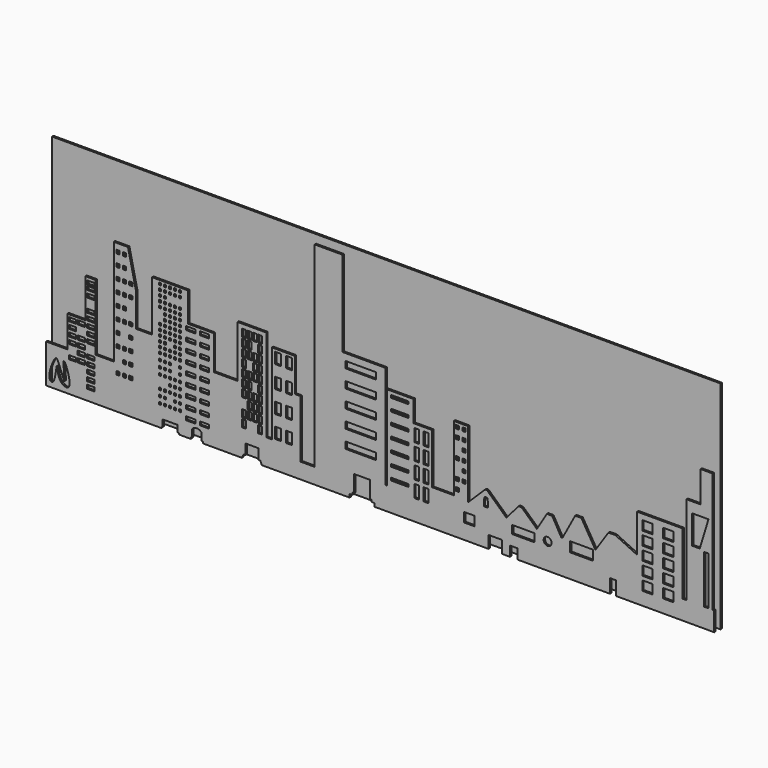
from build123d import *

# Parameters (mm, degrees)
F0_W     = 106.057882309
F0_H     = 53.0289784074
F0_W_2   = 30.3485393524
F0_H_2   = 32.5163006783
F0_W_3   = 133.1057548523
F0_H_3   = 52.0848631859
F0_W_4   = 106.7019701004
F0_H_4   = 55.8841459751
F0_W_5   = 45.7174777985
F0_H_5   = 48.7651824951
F0_W_6   = 57.4026107788
F0_H_6   = 103.5175919533
F0_W_7   = 82.8815102577
F0_H_7   = 156.7766070366
F0_W_8   = 430.9868663549
F0_H_8   = 94.4404602051
F0_W_9   = 149.8684883118
F0_H_9   = 134.093016386
F0_W_10  = 65.5418634415
F0_H_10  = 180.8955073357
F0_W_11  = 249.9276399612
F0_H_11  = 37.1180176735
F0_W_12  = 45.1661348343
F0_H_12  = 48.2810139656
F0_W_13  = 319.1833496094
F0_H_13  = 116.066634655
F0_W_14  = 149.1322517395
F0_H_14  = 133.4340721369
F0_R     = 57.1283266998
F0_W_15  = 327.2154331207
F0_H_15  = 141.2975788116
F0_W_16  = 65.1669502258
F0_H_16  = 692.0295953751
F1_DEPTH = 25.4
F4_DEPTH = 12.7


# Not quite as in the source:
# - a feature names something its author has since deleted; it is built from what else it names


with BuildPart() as f1:
    # F0 (on Front) → F1 (new body)
    with BuildSketch(Plane.XZ):
        with BuildLine():
            Line((-4050, -267.8987085819), (-4050, -823.1540341105))
            Line((-4050, -823.1540341105), (-2398.3292579651, -823.1540341105))
            Line((-2398.3292579651, -823.1540341105), (-2398.3292579651, -805.6496977806))
            Line((-2398.3292579651, -805.6496977806), (-2379.4989585876, -805.6496977806))
            Line((-2379.4989585876, -805.6496977806), (-2379.4989585876, -707.0814371109))
            Line((-2379.4989585876, -707.0814371109), (-2165.6568050385, -707.0814371109))
            Line((-2165.6568050385, -707.0814371109), (-2165.6568050385, -805.6496977806))
            Line((-2165.6568050385, -805.6496977806), (-2146.826505661, -805.6496977806))
            Line((-2146.826505661, -805.6496977806), (-2146.826505661, -823.1540341105))
            Line((-2146.826505661, -823.1540341105), (-1975.0509262085, -823.1540341105))
            Line((-1975.0509262085, -823.1540341105), (-1975.0509262085, -798.1595396996))
            Line((-1975.0509262085, -798.1595396996), (-1956.2240839005, -798.1595396996))
            Line((-1956.2240839005, -798.1595396996), (-1956.2240839005, -691.64955616))
            ThreePointArc((-1956.2240839005, -691.64955616), (-1888.9850974083, -660.7239747575), (-1821.7461109161, -691.64955616))
            Line((-1821.7461109161, -691.64955616), (-1821.7461109161, -798.1595396996))
            Line((-1821.7461109161, -798.1595396996), (-1802.9192686081, -798.1595396996))
            Line((-1802.9192686081, -798.1595396996), (-1802.9192686081, -823.1540341105))
            Line((-1802.9192686081, -823.1540341105), (-1242.5245046616, -823.1540341105))
            Line((-1242.5245046616, -823.1540341105), (-1218.6781167984, -771.0908651352))
            Line((-1218.6781167984, -771.0908651352), (-1190.6187534332, -771.0908651352))
            Line((-1190.6187534332, -771.0908651352), (-1190.6187534332, -624.5583295822))
            Line((-1190.6187534332, -624.5583295822), (-1098.9642441273, -624.5583295822))
            Line((-1098.9642441273, -624.5583295822), (-1007.3097348213, -624.5583295822))
            Line((-1007.3097348213, -624.5583295822), (-1007.3097348213, -771.0908651352))
            Line((-1007.3097348213, -771.0908651352), (-979.2503714561, -771.0908651352))
            Line((-979.2503714561, -771.0908651352), (-955.403983593, -823.1540341105))
            Line((-955.403983593, -823.1540341105), (-200, -823.1540341105))
            Line((-200, -823.1540341105), (200, -823.1540341105))
            Line((200, -823.1540341105), (300.7671995602, -823.1540341105))
            Line((300.7671995602, -823.1540341105), (302.6098906994, -776.0580182076))
            Line((302.6098906994, -776.0580182076), (341.7147696018, -776.0580182076))
            Line((341.7147696018, -776.0580182076), (341.7147696018, -745.5047369003))
            Line((341.7147696018, -745.5047369003), (365.1579022408, -745.5047369003))
            Line((365.1579022408, -745.5047369003), (365.1579022408, -503.856420517))
            Line((365.1579022408, -503.856420517), (593.2507812977, -503.856420517))
            Line((593.2507812977, -503.856420517), (593.2507812977, -745.5047369003))
            Line((593.2507812977, -745.5047369003), (616.6939139366, -745.5047369003))
            Line((616.6939139366, -745.5047369003), (616.6939139366, -776.0580182076))
            Line((616.6939139366, -776.0580182076), (655.7987928391, -776.0580182076))
            Line((655.7987928391, -776.0580182076), (657.6414839782, -823.1540341105))
            Line((657.6414839782, -823.1540341105), (2292.0085966587, -823.1540341105))
            Line((2292.0085966587, -823.1540341105), (2292.0085966587, -646.2127566338))
            Line((2292.0085966587, -646.2127566338), (2486.2071405573, -646.2127566338))
            Line((2486.2071405573, -646.2127566338), (2486.2071405573, -823.1540341105))
            Line((2486.2071405573, -823.1540341105), (2601.8533289433, -823.1540341105))
            Line((2601.8533289433, -823.1540341105), (2601.8533289433, -680.1304221153))
            Line((2601.8533289433, -680.1304221153), (2712.2828543186, -680.1304221153))
            Line((2712.2828543186, -680.1304221153), (2712.2828543186, -823.1540341105))
            Line((2712.2828543186, -823.1540341105), (4036.196231842, -823.1540341105))
            Line((4036.196231842, -823.1540341105), (4036.196231842, -625.0136494637))
            Line((4036.196231842, -625.0136494637), (4124.2990493774, -625.0136494637))
            Line((4124.2990493774, -625.0136494637), (4124.2990493774, -823.1540341105))
            Line((4124.2990493774, -823.1540341105), (5530, -823.1540341105))
            Line((5530, -823.1540341105), (5530, -547.2885370255))
            Line((5530, -547.2885370255), (5506.386756897, -547.2885370255))
            Line((5506.386756897, -547.2885370255), (5506.386756897, 1173.7429499626))
            Line((5506.386756897, 1173.7429499626), (5332.763671875, 1173.7429499626))
            Line((5332.763671875, 1173.7429499626), (5332.1881294251, 726.7968654633))
            Line((5332.1881294251, 726.7968654633), (5132.0977210999, 726.7968654633))
            Line((5132.0977210999, 726.7968654633), (5132.0977210999, -547.2885370255))
            Line((5132.0977210999, -547.2885370255), (5078.1888961792, -547.2885370255))
            Line((5078.1888961792, -547.2885370255), (5078.1888961792, 339.9310410023))
            Line((5078.1888961792, 339.9310410023), (4426.2585639954, 339.9310410023))
            Line((4426.2585639954, 339.9310410023), (4426.2585639954, -206.2637656927))
            Line((4426.2585639954, -206.2637656927), (4106.8322555828, -55.5771386986))
            Line((4106.8322555828, -55.5771386986), (4011.697769165, -60.2504573762))
            Line((4011.697769165, -60.2504573762), (3826.6596794128, -337.2659981251))
            Line((3826.6596794128, -337.2659981251), (3624.871164403, 0))
            Line((3624.871164403, 0), (3536.6790159997, 0))
            Line((3536.6790159997, 0), (3354.7794500447, -337.2186422348))
            Line((3354.7794500447, -337.2186422348), (3336.8639945984, -337.2186422348))
            Line((3336.8639945984, -337.2186422348), (3205.3269538862, -108.8699400425))
            Line((3205.3269538862, -108.8699400425), (3130.6440830231, -108.8699400425))
            Line((3130.6440830231, -108.8699400425), (2987.9386425018, -346.1197912693))
            Line((2987.9386425018, -346.1197912693), (2768.6786679977, -144.6304917336))
            Line((2768.6786679977, -144.6304917336), (2725.0745135728, -144.6304917336))
            Line((2725.0745135728, -144.6304917336), (2549.5419299318, -345.8707353657))
            Line((2549.5419299318, -345.8707353657), (2273.8852819125, -90.167529881))
            Line((2273.8852819125, -90.167529881), (2244.2018143316, -90.167529881))
            Line((2244.2018143316, -90.167529881), (2001.464086771, -329.9159508997))
            Line((2001.464086771, -329.9159508997), (2001.464086771, 630.3516030312))
            Line((2001.464086771, 630.3516030312), (1796.4037881776, 630.3516030312))
            Line((1796.4037881776, 630.3516030312), (1796.4037881776, -308.0070912838))
            Line((1796.4037881776, -308.0070912838), (1485.8823597431, -308.0070912838))
            Line((1485.8823597431, -308.0070912838), (1485.8823597431, 413.8072431087))
            Line((1485.8823597431, 413.8072431087), (1218.7330305576, 413.8072431087))
            Line((1218.7330305576, 413.8072431087), (1218.7330305576, 718.4568047523))
            Line((1218.7330305576, 718.4568047523), (840.5962586403, 718.4568047523))
            Line((840.5962586403, 718.4568047523), (840.5962586403, -498.1889128685))
            Line((840.5962586403, -498.1889128685), (819.9257850647, -498.1889128685))
            Line((819.9257850647, -498.1889128685), (819.9257850647, 718.4568047523))
            Line((819.9257850647, 718.4568047523), (819.9257850647, 981.3694953918))
            Line((819.9257850647, 981.3694953918), (200, 981.3694953918))
            Line((200, 981.3694953918), (200, 2209.0940475464))
            Line((200, 2209.0940475464), (-200, 2209.0940475464))
            Line((-200, 2209.0940475464), (-200, -598.6170768738))
            Line((-200, -598.6170768738), (-402.6772975922, -598.6170768738))
            Line((-402.6772975922, -598.6170768738), (-402.6772975922, 228.1788140535))
            Line((-402.6772975922, 228.1788140535), (-484.4234585762, 228.1788140535))
            Line((-484.4234585762, 228.1788140535), (-484.4234585762, 709.7859978676))
            Line((-484.4234585762, 709.7859978676), (-812.3204112053, 709.7859978676))
            Line((-812.3204112053, 709.7859978676), (-812.3204112053, -451.631128788))
            Line((-812.3204112053, -451.631128788), (-892.2652602196, -451.631128788))
            Line((-892.2652602196, -451.631128788), (-892.2652602196, 871.2424039841))
            Line((-892.2652602196, 871.2424039841), (-1305.663228035, 871.2424039841))
            Line((-1305.663228035, 871.2424039841), (-1305.663228035, 127.1261125803))
            Line((-1305.663228035, 127.1261125803), (-1645.5682516098, 127.1261125803))
            Line((-1645.5682516098, 127.1261125803), (-1645.5682516098, 617.8794503212))
            Line((-1645.5682516098, 617.8794503212), (-2016.7036056519, 617.8794503212))
            Line((-2016.7036056519, 617.8794503212), (-2016.7036056519, 1037.7280712128))
            Line((-2016.7036056519, 1037.7280712128), (-2529.8598766327, 1037.7280712128))
            Line((-2529.8598766327, 1037.7280712128), (-2529.8598766327, 311.6183876991))
            Line((-2529.8598766327, 311.6183876991), (-2762.8433704376, 311.6183876991))
            Line((-2762.8433704376, 311.6183876991), (-2762.8433704376, 799.4017601013))
            Line((-2762.8433704376, 799.4017601013), (-2875.7593631744, 1305.8730363846))
            Line((-2875.7593631744, 1305.8730363846), (-3079.5800685883, 1305.8730363846))
            Line((-3079.5800685883, 1305.8730363846), (-3079.5800685883, -205.8582752943))
            Line((-3079.5800685883, -205.8582752943), (-3342.520570755, -205.8582752943))
            Line((-3342.520570755, -205.8582752943), (-3342.520570755, 739.0350699425))
            Line((-3342.520570755, 739.0350699425), (-3487.3390197754, 739.0350699425))
            Line((-3487.3390197754, 739.0350699425), (-3487.3390197754, 182.2456717491))
            Line((-3487.3390197754, 182.2456717491), (-3744.5102214813, 182.2456717491))
            Line((-3744.5102214813, 182.2456717491), (-3744.5102214813, -267.8987085819))
            Line((-3744.5102214813, -267.8987085819), (-4050, -267.8987085819))
        make_face()
        with BuildLine():
            add(Edge.make_bspline(
                [(-3999.0003108978, -718.5704708099), (-4017.5809404887, -648.1756687185), (-3939.2137069789, -434.2497174078), (-3874.5316623853, -420.5607068995), (-3741.7169424986, -885.2751666982), (-3823.6352453126, -392.4715945569), (-3756.0812047479, -467.0202234965), (-3655.1406239686, -799.785591942), (-3886.5709094027, -724.3440767086), (-3894.1614574012, -392.9639347832), (-3921.3003883476, -791.6671997818), (-3990.7973827964, -749.6481852354), (-3999.0003108978, -718.5704708099)],
                knots=[0, 0, 0, 0, 0.1356772704, 0.1835386764, 0.3131783676, 0.4398985618, 0.4871889594, 0.622511957, 0.7147805439, 0.8199131102, 0.940101551, 1, 1, 1, 1], degree=3))
        make_face(mode=Mode.SUBTRACT)
        with Locations((-3411.3100767136, -647.3052653968)):
            Rectangle(F0_W, F0_H, mode=Mode.SUBTRACT)
        with Locations((-3411.3100767136, -551.3052653968)):
            Rectangle(F0_W, F0_H, mode=Mode.SUBTRACT)
        with Locations((-2418.0961053085, -517.2643567324)):
            Rectangle(F0_W_2, F0_H_2, mode=Mode.SUBTRACT)
        with Locations((-2345.7061053085, -517.2643567324)):
            Rectangle(F0_W_2, F0_H_2, mode=Mode.SUBTRACT)
        with Locations((-2273.3161053085, -517.2643567324)):
            Rectangle(F0_W_2, F0_H_2, mode=Mode.SUBTRACT)
        with Locations((-1977.4153232574, -583.5021812153)):
            Rectangle(F0_W_3, F0_H_3, mode=Mode.SUBTRACT)
        with Locations((-2200.9261053085, -517.2643567324)):
            Rectangle(F0_W_2, F0_H_2, mode=Mode.SUBTRACT)
        with Locations((-2128.5361053085, -517.2643567324)):
            Rectangle(F0_W_2, F0_H_2, mode=Mode.SUBTRACT)
        with Locations((-1779.2953232574, -583.5021812153)):
            Rectangle(F0_W_3, F0_H_3, mode=Mode.SUBTRACT)
        with Locations((-3671.4545488358, -359.3052653968)):
            Rectangle(F0_W, F0_H, mode=Mode.SUBTRACT)
        with Locations((-3542.9670214653, -357.877681613)):
            Rectangle(F0_W_4, F0_H_4, mode=Mode.SUBTRACT)
        with Locations((-3411.3100767136, -455.3052653968)):
            Rectangle(F0_W, F0_H, mode=Mode.SUBTRACT)
        with Locations((-3411.3100767136, -359.3052653968)):
            Rectangle(F0_W, F0_H, mode=Mode.SUBTRACT)
        with Locations((-3016.9705152512, -334.5595884323)):
            Rectangle(F0_W_5, F0_H_5, mode=Mode.SUBTRACT)
        with Locations((-2926.9705152512, -334.5595884323)):
            Rectangle(F0_W_5, F0_H_5, mode=Mode.SUBTRACT)
        with Locations((-3542.9670214653, -261.877681613)):
            Rectangle(F0_W_4, F0_H_4, mode=Mode.SUBTRACT)
        with Locations((-3671.4545488358, -167.3052653968)):
            Rectangle(F0_W, F0_H, mode=Mode.SUBTRACT)
        with Locations((-3542.9670214653, -165.877681613)):
            Rectangle(F0_W_4, F0_H_4, mode=Mode.SUBTRACT)
        with Locations((-3411.3100767136, -263.3052653968)):
            Rectangle(F0_W, F0_H, mode=Mode.SUBTRACT)
        with Locations((-2926.9705152512, -164.5595884323)):
            Rectangle(F0_W_5, F0_H_5, mode=Mode.SUBTRACT)
        with Locations((-2418.0961053085, -426.2643567324)):
            Rectangle(F0_W_2, F0_H_2, mode=Mode.SUBTRACT)
        with Locations((-2345.7061053085, -426.2643567324)):
            Rectangle(F0_W_2, F0_H_2, mode=Mode.SUBTRACT)
        with Locations((-2836.9705152512, -334.5595884323)):
            Rectangle(F0_W_5, F0_H_5, mode=Mode.SUBTRACT)
        with Locations((-2418.0961053085, -335.2643567324)):
            Rectangle(F0_W_2, F0_H_2, mode=Mode.SUBTRACT)
        with Locations((-2345.7061053085, -335.2643567324)):
            Rectangle(F0_W_2, F0_H_2, mode=Mode.SUBTRACT)
        with Locations((-2273.3161053085, -335.2643567324)):
            Rectangle(F0_W_2, F0_H_2, mode=Mode.SUBTRACT)
        with Locations((-2200.9261053085, -426.2643567324)):
            Rectangle(F0_W_2, F0_H_2, mode=Mode.SUBTRACT)
        with Locations((-2128.5361053085, -426.2643567324)):
            Rectangle(F0_W_2, F0_H_2, mode=Mode.SUBTRACT)
        with Locations((-1977.4153232574, -441.2621812153)):
            Rectangle(F0_W_3, F0_H_3, mode=Mode.SUBTRACT)
        with Locations((-1779.2953232574, -441.2621812153)):
            Rectangle(F0_W_3, F0_H_3, mode=Mode.SUBTRACT)
        with Locations((-2200.9261053085, -335.2643567324)):
            Rectangle(F0_W_2, F0_H_2, mode=Mode.SUBTRACT)
        with Locations((-2128.5361053085, -335.2643567324)):
            Rectangle(F0_W_2, F0_H_2, mode=Mode.SUBTRACT)
        with Locations((-2273.3161053085, -244.2643567324)):
            Rectangle(F0_W_2, F0_H_2, mode=Mode.SUBTRACT)
        with Locations((-2836.9705152512, -164.5595884323)):
            Rectangle(F0_W_5, F0_H_5, mode=Mode.SUBTRACT)
        with Locations((-2418.0961053085, -153.2643567324)):
            Rectangle(F0_W_2, F0_H_2, mode=Mode.SUBTRACT)
        with Locations((-2345.7061053085, -153.2643567324)):
            Rectangle(F0_W_2, F0_H_2, mode=Mode.SUBTRACT)
        with Locations((-2273.3161053085, -153.2643567324)):
            Rectangle(F0_W_2, F0_H_2, mode=Mode.SUBTRACT)
        with Locations((-1977.4153232574, -299.0221812153)):
            Rectangle(F0_W_3, F0_H_3, mode=Mode.SUBTRACT)
        with Locations((-2200.9261053085, -244.2643567324)):
            Rectangle(F0_W_2, F0_H_2, mode=Mode.SUBTRACT)
        with Locations((-2128.5361053085, -244.2643567324)):
            Rectangle(F0_W_2, F0_H_2, mode=Mode.SUBTRACT)
        with Locations((-1779.2953232574, -299.0221812153)):
            Rectangle(F0_W_3, F0_H_3, mode=Mode.SUBTRACT)
        with Locations((-2200.9261053085, -153.2643567324)):
            Rectangle(F0_W_2, F0_H_2, mode=Mode.SUBTRACT)
        with Locations((-2128.5361053085, -153.2643567324)):
            Rectangle(F0_W_2, F0_H_2, mode=Mode.SUBTRACT)
        with Locations((-1977.4153232574, -156.7821812153)):
            Rectangle(F0_W_3, F0_H_3, mode=Mode.SUBTRACT)
        with Locations((-1779.2953232574, -156.7821812153)):
            Rectangle(F0_W_3, F0_H_3, mode=Mode.SUBTRACT)
        with Locations((-1210.2817296982, -385.5909936428)):
            Rectangle(F0_W_6, F0_H_6, mode=Mode.SUBTRACT)
        with Locations((-981.6817296982, -385.5909936428)):
            Rectangle(F0_W_6, F0_H_6, mode=Mode.SUBTRACT)
        with Locations((-724.9703705311, -352.009317522)):
            Rectangle(F0_W_7, F0_H_7, mode=Mode.SUBTRACT)
        with Locations((-564.9503705311, -352.009317522)):
            Rectangle(F0_W_7, F0_H_7, mode=Mode.SUBTRACT)
        with Locations((-1210.2817296982, -258.5909936428)):
            Rectangle(F0_W_6, F0_H_6, mode=Mode.SUBTRACT)
        with Locations((-1134.0817296982, -258.5909936428)):
            Rectangle(F0_W_6, F0_H_6, mode=Mode.SUBTRACT)
        with Locations((-1057.8817296982, -258.5909936428)):
            Rectangle(F0_W_6, F0_H_6, mode=Mode.SUBTRACT)
        with Locations((-1134.0817296982, -131.5909936428)):
            Rectangle(F0_W_6, F0_H_6, mode=Mode.SUBTRACT)
        with Locations((-1057.8817296982, -131.5909936428)):
            Rectangle(F0_W_6, F0_H_6, mode=Mode.SUBTRACT)
        with Locations((-981.6817296982, -258.5909936428)):
            Rectangle(F0_W_6, F0_H_6, mode=Mode.SUBTRACT)
        with Locations((-981.6817296982, -131.5909936428)):
            Rectangle(F0_W_6, F0_H_6, mode=Mode.SUBTRACT)
        with Locations((461.999244988, -180.1629338264)):
            Rectangle(F0_W_8, F0_H_8, mode=Mode.SUBTRACT)
        with Locations((-3671.4545488358, -71.3052653968)):
            Rectangle(F0_W, F0_H, mode=Mode.SUBTRACT)
        with Locations((-3542.9670214653, -69.877681613)):
            Rectangle(F0_W_4, F0_H_4, mode=Mode.SUBTRACT)
        with Locations((-3671.4545488358, 24.6947346032)):
            Rectangle(F0_W, F0_H, mode=Mode.SUBTRACT)
        with Locations((-3411.3100767136, -71.3052653968)):
            Rectangle(F0_W, F0_H, mode=Mode.SUBTRACT)
        with Locations((-3411.3100767136, 24.6947346032)):
            Rectangle(F0_W, F0_H, mode=Mode.SUBTRACT)
        with Locations((-3016.9705152512, 5.4404115677)):
            Rectangle(F0_W_5, F0_H_5, mode=Mode.SUBTRACT)
        with Locations((-2926.9705152512, 5.4404115677)):
            Rectangle(F0_W_5, F0_H_5, mode=Mode.SUBTRACT)
        with Locations((-3671.4545488358, 120.6947346032)):
            Rectangle(F0_W, F0_H, mode=Mode.SUBTRACT)
        with Locations((-3542.9670214653, 122.122318387)):
            Rectangle(F0_W_4, F0_H_4, mode=Mode.SUBTRACT)
        with Locations((-3411.3100767136, 120.6947346032)):
            Rectangle(F0_W, F0_H, mode=Mode.SUBTRACT)
        with Locations((-3016.9705152512, 175.4404115677)):
            Rectangle(F0_W_5, F0_H_5, mode=Mode.SUBTRACT)
        with Locations((-3411.3100767136, 216.6947346032)):
            Rectangle(F0_W, F0_H, mode=Mode.SUBTRACT)
        with Locations((-2418.0961053085, -62.2643567324)):
            Rectangle(F0_W_2, F0_H_2, mode=Mode.SUBTRACT)
        with Locations((-2345.7061053085, -62.2643567324)):
            Rectangle(F0_W_2, F0_H_2, mode=Mode.SUBTRACT)
        with Locations((-2273.3161053085, -62.2643567324)):
            Rectangle(F0_W_2, F0_H_2, mode=Mode.SUBTRACT)
        with Locations((-2836.9705152512, 5.4404115677)):
            Rectangle(F0_W_5, F0_H_5, mode=Mode.SUBTRACT)
        with Locations((-2418.0961053085, 28.7356432676)):
            Rectangle(F0_W_2, F0_H_2, mode=Mode.SUBTRACT)
        with Locations((-2345.7061053085, 28.7356432676)):
            Rectangle(F0_W_2, F0_H_2, mode=Mode.SUBTRACT)
        with Locations((-2273.3161053085, 28.7356432676)):
            Rectangle(F0_W_2, F0_H_2, mode=Mode.SUBTRACT)
        with Locations((-2128.5361053085, -62.2643567324)):
            Rectangle(F0_W_2, F0_H_2, mode=Mode.SUBTRACT)
        with Locations((-2128.5361053085, 28.7356432676)):
            Rectangle(F0_W_2, F0_H_2, mode=Mode.SUBTRACT)
        with Locations((-1977.4153232574, -14.5421812153)):
            Rectangle(F0_W_3, F0_H_3, mode=Mode.SUBTRACT)
        with Locations((-1779.2953232574, -14.5421812153)):
            Rectangle(F0_W_3, F0_H_3, mode=Mode.SUBTRACT)
        with Locations((-2836.9705152512, 175.4404115677)):
            Rectangle(F0_W_5, F0_H_5, mode=Mode.SUBTRACT)
        with Locations((-2418.0961053085, 119.7356432676)):
            Rectangle(F0_W_2, F0_H_2, mode=Mode.SUBTRACT)
        with Locations((-2345.7061053085, 119.7356432676)):
            Rectangle(F0_W_2, F0_H_2, mode=Mode.SUBTRACT)
        with Locations((-2273.3161053085, 119.7356432676)):
            Rectangle(F0_W_2, F0_H_2, mode=Mode.SUBTRACT)
        with Locations((-2418.0961053085, 192.1256432676)):
            Rectangle(F0_W_2, F0_H_2, mode=Mode.SUBTRACT)
        with Locations((-2345.7061053085, 192.1256432676)):
            Rectangle(F0_W_2, F0_H_2, mode=Mode.SUBTRACT)
        with Locations((-2273.3161053085, 192.1256432676)):
            Rectangle(F0_W_2, F0_H_2, mode=Mode.SUBTRACT)
        with Locations((-2418.0961053085, 264.5156432676)):
            Rectangle(F0_W_2, F0_H_2, mode=Mode.SUBTRACT)
        with Locations((-2345.7061053085, 264.5156432676)):
            Rectangle(F0_W_2, F0_H_2, mode=Mode.SUBTRACT)
        with Locations((-2200.9261053085, 119.7356432676)):
            Rectangle(F0_W_2, F0_H_2, mode=Mode.SUBTRACT)
        with Locations((-2128.5361053085, 119.7356432676)):
            Rectangle(F0_W_2, F0_H_2, mode=Mode.SUBTRACT)
        with Locations((-1977.4153232574, 127.6978187847)):
            Rectangle(F0_W_3, F0_H_3, mode=Mode.SUBTRACT)
        with Locations((-1779.2953232574, 127.6978187847)):
            Rectangle(F0_W_3, F0_H_3, mode=Mode.SUBTRACT)
        with Locations((-2200.9261053085, 192.1256432676)):
            Rectangle(F0_W_2, F0_H_2, mode=Mode.SUBTRACT)
        with Locations((-2128.5361053085, 192.1256432676)):
            Rectangle(F0_W_2, F0_H_2, mode=Mode.SUBTRACT)
        with Locations((-2200.9261053085, 264.5156432676)):
            Rectangle(F0_W_2, F0_H_2, mode=Mode.SUBTRACT)
        with Locations((-2128.5361053085, 264.5156432676)):
            Rectangle(F0_W_2, F0_H_2, mode=Mode.SUBTRACT)
        with Locations((-1977.4153232574, 269.9378187847)):
            Rectangle(F0_W_3, F0_H_3, mode=Mode.SUBTRACT)
        with Locations((-1779.2953232574, 269.9378187847)):
            Rectangle(F0_W_3, F0_H_3, mode=Mode.SUBTRACT)
        with Locations((-3411.3100767136, 312.6947346032)):
            Rectangle(F0_W, F0_H, mode=Mode.SUBTRACT)
        with Locations((-3016.9705152512, 345.4404115677)):
            Rectangle(F0_W_5, F0_H_5, mode=Mode.SUBTRACT)
        with Locations((-2926.9705152512, 345.4404115677)):
            Rectangle(F0_W_5, F0_H_5, mode=Mode.SUBTRACT)
        with Locations((-3411.3100767136, 504.6947346032)):
            Rectangle(F0_W, F0_H, mode=Mode.SUBTRACT)
        with Locations((-3016.9705152512, 515.4404115677)):
            Rectangle(F0_W_5, F0_H_5, mode=Mode.SUBTRACT)
        with Locations((-2926.9705152512, 515.4404115677)):
            Rectangle(F0_W_5, F0_H_5, mode=Mode.SUBTRACT)
        with Locations((-3411.3100767136, 600.6947346032)):
            Rectangle(F0_W, F0_H, mode=Mode.SUBTRACT)
        with Locations((-2836.9705152512, 345.4404115677)):
            Rectangle(F0_W_5, F0_H_5, mode=Mode.SUBTRACT)
        with Locations((-2418.0961053085, 336.9056432676)):
            Rectangle(F0_W_2, F0_H_2, mode=Mode.SUBTRACT)
        with Locations((-2345.7061053085, 336.9056432676)):
            Rectangle(F0_W_2, F0_H_2, mode=Mode.SUBTRACT)
        with Locations((-2273.3161053085, 336.9056432676)):
            Rectangle(F0_W_2, F0_H_2, mode=Mode.SUBTRACT)
        with Locations((-2418.0961053085, 409.2956432676)):
            Rectangle(F0_W_2, F0_H_2, mode=Mode.SUBTRACT)
        with Locations((-2345.7061053085, 409.2956432676)):
            Rectangle(F0_W_2, F0_H_2, mode=Mode.SUBTRACT)
        with Locations((-2273.3161053085, 409.2956432676)):
            Rectangle(F0_W_2, F0_H_2, mode=Mode.SUBTRACT)
        with Locations((-2200.9261053085, 336.9056432676)):
            Rectangle(F0_W_2, F0_H_2, mode=Mode.SUBTRACT)
        with Locations((-2128.5361053085, 336.9056432676)):
            Rectangle(F0_W_2, F0_H_2, mode=Mode.SUBTRACT)
        with Locations((-2200.9261053085, 409.2956432676)):
            Rectangle(F0_W_2, F0_H_2, mode=Mode.SUBTRACT)
        with Locations((-2128.5361053085, 409.2956432676)):
            Rectangle(F0_W_2, F0_H_2, mode=Mode.SUBTRACT)
        with Locations((-1977.4153232574, 412.1778187847)):
            Rectangle(F0_W_3, F0_H_3, mode=Mode.SUBTRACT)
        with Locations((-1779.2953232574, 412.1778187847)):
            Rectangle(F0_W_3, F0_H_3, mode=Mode.SUBTRACT)
        with Locations((-2418.0961053085, 481.6856432676)):
            Rectangle(F0_W_2, F0_H_2, mode=Mode.SUBTRACT)
        with Locations((-2345.7061053085, 481.6856432676)):
            Rectangle(F0_W_2, F0_H_2, mode=Mode.SUBTRACT)
        with Locations((-2273.3161053085, 481.6856432676)):
            Rectangle(F0_W_2, F0_H_2, mode=Mode.SUBTRACT)
        with Locations((-2345.7061053085, 554.0756432676)):
            Rectangle(F0_W_2, F0_H_2, mode=Mode.SUBTRACT)
        with Locations((-2273.3161053085, 554.0756432676)):
            Rectangle(F0_W_2, F0_H_2, mode=Mode.SUBTRACT)
        with Locations((-2345.7061053085, 626.4656432676)):
            Rectangle(F0_W_2, F0_H_2, mode=Mode.SUBTRACT)
        with Locations((-2273.3161053085, 626.4656432676)):
            Rectangle(F0_W_2, F0_H_2, mode=Mode.SUBTRACT)
        with Locations((-2200.9261053085, 481.6856432676)):
            Rectangle(F0_W_2, F0_H_2, mode=Mode.SUBTRACT)
        with Locations((-2128.5361053085, 481.6856432676)):
            Rectangle(F0_W_2, F0_H_2, mode=Mode.SUBTRACT)
        with Locations((-2200.9261053085, 554.0756432676)):
            Rectangle(F0_W_2, F0_H_2, mode=Mode.SUBTRACT)
        with Locations((-2128.5361053085, 554.0756432676)):
            Rectangle(F0_W_2, F0_H_2, mode=Mode.SUBTRACT)
        with Locations((-1977.4153232574, 554.4178187847)):
            Rectangle(F0_W_3, F0_H_3, mode=Mode.SUBTRACT)
        with Locations((-1779.2953232574, 554.4178187847)):
            Rectangle(F0_W_3, F0_H_3, mode=Mode.SUBTRACT)
        with Locations((-2200.9261053085, 626.4656432676)):
            Rectangle(F0_W_2, F0_H_2, mode=Mode.SUBTRACT)
        with Locations((-2128.5361053085, 626.4656432676)):
            Rectangle(F0_W_2, F0_H_2, mode=Mode.SUBTRACT)
        with Locations((-1210.2817296982, -4.5909936428)):
            Rectangle(F0_W_6, F0_H_6, mode=Mode.SUBTRACT)
        with Locations((-1134.0817296982, -4.5909936428)):
            Rectangle(F0_W_6, F0_H_6, mode=Mode.SUBTRACT)
        with Locations((-1057.8817296982, -4.5909936428)):
            Rectangle(F0_W_6, F0_H_6, mode=Mode.SUBTRACT)
        with Locations((-724.9703705311, -37.049317522)):
            Rectangle(F0_W_7, F0_H_7, mode=Mode.SUBTRACT)
        with Locations((-564.9503705311, -37.049317522)):
            Rectangle(F0_W_7, F0_H_7, mode=Mode.SUBTRACT)
        with Locations((-981.6817296982, -4.5909936428)):
            Rectangle(F0_W_6, F0_H_6, mode=Mode.SUBTRACT)
        with Locations((-1210.2817296982, 122.4090063572)):
            Rectangle(F0_W_6, F0_H_6, mode=Mode.SUBTRACT)
        with Locations((-1134.0817296982, 122.4090063572)):
            Rectangle(F0_W_6, F0_H_6, mode=Mode.SUBTRACT)
        with Locations((-1210.2817296982, 249.4090063572)):
            Rectangle(F0_W_6, F0_H_6, mode=Mode.SUBTRACT)
        with Locations((-1134.0817296982, 249.4090063572)):
            Rectangle(F0_W_6, F0_H_6, mode=Mode.SUBTRACT)
        with Locations((-1057.8817296982, 249.4090063572)):
            Rectangle(F0_W_6, F0_H_6, mode=Mode.SUBTRACT)
        with Locations((-981.6817296982, 122.4090063572)):
            Rectangle(F0_W_6, F0_H_6, mode=Mode.SUBTRACT)
        with Locations((-981.6817296982, 249.4090063572)):
            Rectangle(F0_W_6, F0_H_6, mode=Mode.SUBTRACT)
        with Locations((461.999244988, 73.8370661736)):
            Rectangle(F0_W_8, F0_H_8, mode=Mode.SUBTRACT)
        with Locations((-1210.2817296982, 376.4090063572)):
            Rectangle(F0_W_6, F0_H_6, mode=Mode.SUBTRACT)
        with Locations((-1057.8817296982, 376.4090063572)):
            Rectangle(F0_W_6, F0_H_6, mode=Mode.SUBTRACT)
        with Locations((-724.9703705311, 277.910682478)):
            Rectangle(F0_W_7, F0_H_7, mode=Mode.SUBTRACT)
        with Locations((-564.9503705311, 277.910682478)):
            Rectangle(F0_W_7, F0_H_7, mode=Mode.SUBTRACT)
        with Locations((-981.6817296982, 376.4090063572)):
            Rectangle(F0_W_6, F0_H_6, mode=Mode.SUBTRACT)
        with Locations((-1210.2817296982, 503.4090063572)):
            Rectangle(F0_W_6, F0_H_6, mode=Mode.SUBTRACT)
        with Locations((-1134.0817296982, 503.4090063572)):
            Rectangle(F0_W_6, F0_H_6, mode=Mode.SUBTRACT)
        with Locations((-1057.8817296982, 503.4090063572)):
            Rectangle(F0_W_6, F0_H_6, mode=Mode.SUBTRACT)
        with Locations((-1210.2817296982, 630.4090063572)):
            Rectangle(F0_W_6, F0_H_6, mode=Mode.SUBTRACT)
        with Locations((-1134.0817296982, 630.4090063572)):
            Rectangle(F0_W_6, F0_H_6, mode=Mode.SUBTRACT)
        with Locations((-981.6817296982, 503.4090063572)):
            Rectangle(F0_W_6, F0_H_6, mode=Mode.SUBTRACT)
        with Locations((-981.6817296982, 630.4090063572)):
            Rectangle(F0_W_6, F0_H_6, mode=Mode.SUBTRACT)
        with Locations((-724.9703705311, 592.870682478)):
            Rectangle(F0_W_7, F0_H_7, mode=Mode.SUBTRACT)
        with Locations((-564.9503705311, 592.870682478)):
            Rectangle(F0_W_7, F0_H_7, mode=Mode.SUBTRACT)
        with Locations((461.999244988, 327.8370661736)):
            Rectangle(F0_W_8, F0_H_8, mode=Mode.SUBTRACT)
        with Locations((461.999244988, 581.8370661736)):
            Rectangle(F0_W_8, F0_H_8, mode=Mode.SUBTRACT)
        with Locations((2018.4049606323, -536.8349701166)):
            Rectangle(F0_W_9, F0_H_9, mode=Mode.SUBTRACT)
        with Locations((1262.2490525246, -436.7391633987)):
            Rectangle(F0_W_10, F0_H_10, mode=Mode.SUBTRACT)
        with Locations((1018.366754055, -396.0775139332)):
            Rectangle(F0_W_11, F0_H_11, mode=Mode.SUBTRACT)
        with Locations((1397.2490525246, -436.7391633987)):
            Rectangle(F0_W_10, F0_H_10, mode=Mode.SUBTRACT)
        with Locations((1018.366754055, -222.0775139332)):
            Rectangle(F0_W_11, F0_H_11, mode=Mode.SUBTRACT)
        with Locations((1262.2490525246, -201.7391633987)):
            Rectangle(F0_W_10, F0_H_10, mode=Mode.SUBTRACT)
        with Locations((1844.8156714439, -218.5361549854)):
            Rectangle(F0_W_12, F0_H_12, mode=Mode.SUBTRACT)
        with Locations((1397.2490525246, -201.7391633987)):
            Rectangle(F0_W_10, F0_H_10, mode=Mode.SUBTRACT)
        with Locations((2793.7183380127, -467.6575362682)):
            Rectangle(F0_W_13, F0_H_13, mode=Mode.SUBTRACT)
        Polygon((2287.0638370514, -306.4538836479), (2225.8064746857, -306.4538836479), (2225.8064746857, -238.7483417988), (2237.5664710999, -182.4237704277), (2256.4351558685, -182.4237704277), (2275.3038406372, -182.4237704277), (2287.0638370514, -238.7483417988), align=None, mode=Mode.SUBTRACT)
        with Locations((4573.7421512604, -567.9705610871)):
            Rectangle(F0_W_14, F0_H_14, mode=Mode.SUBTRACT)
        with Locations((4873.7421512604, -567.9705610871)):
            Rectangle(F0_W_14, F0_H_14, mode=Mode.SUBTRACT)
        with Locations((3141.0386562347, -452.9336839914)):
            Circle(F0_R, mode=Mode.SUBTRACT)
        with Locations((3628.1675100327, -415.6747460365)):
            Rectangle(F0_W_15, F0_H_15, mode=Mode.SUBTRACT)
        with Locations((4573.7421512604, -377.9705610871)):
            Rectangle(F0_W_14, F0_H_14, mode=Mode.SUBTRACT)
        with Locations((4873.7421512604, -377.9705610871)):
            Rectangle(F0_W_14, F0_H_14, mode=Mode.SUBTRACT)
        with Locations((4573.7421512604, -187.9705610871)):
            Rectangle(F0_W_14, F0_H_14, mode=Mode.SUBTRACT)
        with Locations((4873.7421512604, -187.9705610871)):
            Rectangle(F0_W_14, F0_H_14, mode=Mode.SUBTRACT)
        with Locations((5418.8115596771, -201.2737393379)):
            Rectangle(F0_W_16, F0_H_16, mode=Mode.SUBTRACT)
        with Locations((1018.366754055, -48.0775139332)):
            Rectangle(F0_W_11, F0_H_11, mode=Mode.SUBTRACT)
        with Locations((1262.2490525246, 33.2608366013)):
            Rectangle(F0_W_10, F0_H_10, mode=Mode.SUBTRACT)
        with Locations((1844.8156714439, -87.5361549854)):
            Rectangle(F0_W_12, F0_H_12, mode=Mode.SUBTRACT)
        with Locations((1397.2490525246, 33.2608366013)):
            Rectangle(F0_W_10, F0_H_10, mode=Mode.SUBTRACT)
        with Locations((1018.366754055, 125.9224860668)):
            Rectangle(F0_W_11, F0_H_11, mode=Mode.SUBTRACT)
        with Locations((1262.2490525246, 268.2608366013)):
            Rectangle(F0_W_10, F0_H_10, mode=Mode.SUBTRACT)
        with Locations((1844.8156714439, 174.4638450146)):
            Rectangle(F0_W_12, F0_H_12, mode=Mode.SUBTRACT)
        with Locations((1397.2490525246, 268.2608366013)):
            Rectangle(F0_W_10, F0_H_10, mode=Mode.SUBTRACT)
        with Locations((1941.5708184242, -87.5361549854)):
            Rectangle(F0_W_12, F0_H_12, mode=Mode.SUBTRACT)
        with Locations((1941.5708184242, 43.4638450146)):
            Rectangle(F0_W_12, F0_H_12, mode=Mode.SUBTRACT)
        with Locations((1941.5708184242, 174.4638450146)):
            Rectangle(F0_W_12, F0_H_12, mode=Mode.SUBTRACT)
        with Locations((1018.366754055, 299.9224860668)):
            Rectangle(F0_W_11, F0_H_11, mode=Mode.SUBTRACT)
        with Locations((1844.8156714439, 436.4638450146)):
            Rectangle(F0_W_12, F0_H_12, mode=Mode.SUBTRACT)
        with Locations((1018.366754055, 473.9224860668)):
            Rectangle(F0_W_11, F0_H_11, mode=Mode.SUBTRACT)
        with Locations((1018.366754055, 647.9224860668)):
            Rectangle(F0_W_11, F0_H_11, mode=Mode.SUBTRACT)
        with Locations((1844.8156714439, 567.4638450146)):
            Rectangle(F0_W_12, F0_H_12, mode=Mode.SUBTRACT)
        with Locations((1941.5708184242, 305.4638450146)):
            Rectangle(F0_W_12, F0_H_12, mode=Mode.SUBTRACT)
        with Locations((1941.5708184242, 436.4638450146)):
            Rectangle(F0_W_12, F0_H_12, mode=Mode.SUBTRACT)
        with Locations((1941.5708184242, 567.4638450146)):
            Rectangle(F0_W_12, F0_H_12, mode=Mode.SUBTRACT)
        with Locations((4573.7421512604, 2.0294389129)):
            Rectangle(F0_W_14, F0_H_14, mode=Mode.SUBTRACT)
        with Locations((4873.7421512604, 2.0294389129)):
            Rectangle(F0_W_14, F0_H_14, mode=Mode.SUBTRACT)
        with Locations((4573.7421512604, 192.0294389129)):
            Rectangle(F0_W_14, F0_H_14, mode=Mode.SUBTRACT)
        with Locations((4873.7421512604, 192.0294389129)):
            Rectangle(F0_W_14, F0_H_14, mode=Mode.SUBTRACT)
        Polygon((5212.495803833, 576.7448544502), (5447.9417800903, 576.7448544502), (5322.4445699473, 166.2166416645), (5212.495803833, 166.2166416645), align=None, mode=Mode.SUBTRACT)
        with Locations((-3411.3100767136, 669.6265526116)):
            Rectangle(F0_W, F0_H, mode=Mode.SUBTRACT)
        with Locations((-3016.9705152512, 685.4404115677)):
            Rectangle(F0_W_5, F0_H_5, mode=Mode.SUBTRACT)
        with Locations((-2926.9705152512, 685.4404115677)):
            Rectangle(F0_W_5, F0_H_5, mode=Mode.SUBTRACT)
        with Locations((-3016.9705152512, 855.4404115677)):
            Rectangle(F0_W_5, F0_H_5, mode=Mode.SUBTRACT)
        with Locations((-2926.9705152512, 855.4404115677)):
            Rectangle(F0_W_5, F0_H_5, mode=Mode.SUBTRACT)
        with Locations((-3016.9705152512, 1025.4404115677)):
            Rectangle(F0_W_5, F0_H_5, mode=Mode.SUBTRACT)
        with Locations((-2926.9705152512, 1025.4404115677)):
            Rectangle(F0_W_5, F0_H_5, mode=Mode.SUBTRACT)
        with Locations((-2836.9705152512, 685.4404115677)):
            Rectangle(F0_W_5, F0_H_5, mode=Mode.SUBTRACT)
        with Locations((-2418.0961053085, 698.8556432676)):
            Rectangle(F0_W_2, F0_H_2, mode=Mode.SUBTRACT)
        with Locations((-2345.7061053085, 698.8556432676)):
            Rectangle(F0_W_2, F0_H_2, mode=Mode.SUBTRACT)
        with Locations((-2273.3161053085, 698.8556432676)):
            Rectangle(F0_W_2, F0_H_2, mode=Mode.SUBTRACT)
        with Locations((-2418.0961053085, 771.2456432676)):
            Rectangle(F0_W_2, F0_H_2, mode=Mode.SUBTRACT)
        with Locations((-2345.7061053085, 771.2456432676)):
            Rectangle(F0_W_2, F0_H_2, mode=Mode.SUBTRACT)
        with Locations((-2273.3161053085, 771.2456432676)):
            Rectangle(F0_W_2, F0_H_2, mode=Mode.SUBTRACT)
        with Locations((-2418.0961053085, 843.6356432676)):
            Rectangle(F0_W_2, F0_H_2, mode=Mode.SUBTRACT)
        with Locations((-2345.7061053085, 843.6356432676)):
            Rectangle(F0_W_2, F0_H_2, mode=Mode.SUBTRACT)
        with Locations((-2200.9261053085, 698.8556432676)):
            Rectangle(F0_W_2, F0_H_2, mode=Mode.SUBTRACT)
        with Locations((-2128.5361053085, 698.8556432676)):
            Rectangle(F0_W_2, F0_H_2, mode=Mode.SUBTRACT)
        with Locations((-2200.9261053085, 771.2456432676)):
            Rectangle(F0_W_2, F0_H_2, mode=Mode.SUBTRACT)
        with Locations((-2128.5361053085, 771.2456432676)):
            Rectangle(F0_W_2, F0_H_2, mode=Mode.SUBTRACT)
        with Locations((-2836.9705152512, 855.4404115677)):
            Rectangle(F0_W_5, F0_H_5, mode=Mode.SUBTRACT)
        with Locations((-2418.0961053085, 916.0256432676)):
            Rectangle(F0_W_2, F0_H_2, mode=Mode.SUBTRACT)
        with Locations((-2345.7061053085, 916.0256432676)):
            Rectangle(F0_W_2, F0_H_2, mode=Mode.SUBTRACT)
        with Locations((-2273.3161053085, 916.0256432676)):
            Rectangle(F0_W_2, F0_H_2, mode=Mode.SUBTRACT)
        with Locations((-2418.0961053085, 988.4156432676)):
            Rectangle(F0_W_2, F0_H_2, mode=Mode.SUBTRACT)
        with Locations((-2345.7061053085, 988.4156432676)):
            Rectangle(F0_W_2, F0_H_2, mode=Mode.SUBTRACT)
        with Locations((-2273.3161053085, 988.4156432676)):
            Rectangle(F0_W_2, F0_H_2, mode=Mode.SUBTRACT)
        with Locations((-2200.9261053085, 916.0256432676)):
            Rectangle(F0_W_2, F0_H_2, mode=Mode.SUBTRACT)
        with Locations((-2128.5361053085, 916.0256432676)):
            Rectangle(F0_W_2, F0_H_2, mode=Mode.SUBTRACT)
        with Locations((-2200.9261053085, 988.4156432676)):
            Rectangle(F0_W_2, F0_H_2, mode=Mode.SUBTRACT)
        with Locations((-2128.5361053085, 988.4156432676)):
            Rectangle(F0_W_2, F0_H_2, mode=Mode.SUBTRACT)
        with Locations((-3016.9705152512, 1195.4404115677)):
            Rectangle(F0_W_5, F0_H_5, mode=Mode.SUBTRACT)
        with Locations((-2926.9705152512, 1195.4404115677)):
            Rectangle(F0_W_5, F0_H_5, mode=Mode.SUBTRACT)
        with Locations((-1210.2817296982, 757.4090063572)):
            Rectangle(F0_W_6, F0_H_6, mode=Mode.SUBTRACT)
        with Locations((-1134.0817296982, 757.4090063572)):
            Rectangle(F0_W_6, F0_H_6, mode=Mode.SUBTRACT)
        with Locations((-1057.8817296982, 757.4090063572)):
            Rectangle(F0_W_6, F0_H_6, mode=Mode.SUBTRACT)
        with Locations((-981.6817296982, 757.4090063572)):
            Rectangle(F0_W_6, F0_H_6, mode=Mode.SUBTRACT)
        with Locations((461.999244988, 835.8370661736)):
            Rectangle(F0_W_8, F0_H_8, mode=Mode.SUBTRACT)
    extrude(amount=F1_DEPTH)


with BuildPart() as f4:
    # F3 (on offset) → F4 (new body, symmetric)
    with BuildSketch(Plane.XZ.offset(-127)):
        Polygon((-4077.906370163, -850.4594564438), (5508.4722042084, -850.4594564438), (5508.4722042084, 2253.4593343735), (-469.4082140923, 2253.4593343735), (-469.4082140923, 1021.4567184448), (-875.3519058228, 1021.4567184448), (-875.3519058228, 2029.3171405792), (-1211.3053798676, 2029.3171405792), (-1211.3053798676, 1441.3985013962), (-1715.2355909348, 1441.3985013962), (-1715.2355909348, 2253.4593343735), (-2359.1463565826, 2253.4593343735), (-2359.1463565826, 1413.4024381638), (-3122.0405101776, 1413.4024381638), (-3122.0405101776, 1805.3481578827), (-3436.9969367981, 1805.3481578827), (-3436.9969367981, 1084.4479799271), (-4077.906370163, 1084.4479799271), align=None)
        Polygon((-4077.906370163, 2253.4593343735), (-4077.906370163, 1084.4479799271), (-3436.9969367981, 1084.4479799271), (-3436.9969367981, 1805.3481578827), (-3122.0405101776, 1805.3481578827), (-3122.0405101776, 1413.4024381638), (-2359.1463565826, 1413.4024381638), (-2359.1463565826, 2253.4593343735), align=None)
        Polygon((-469.4082140923, 1021.4567184448), (-469.4082140923, 2253.4593343735), (-1715.2355909348, 2253.4593343735), (-1715.2355909348, 1441.3985013962), (-1211.3053798676, 1441.3985013962), (-1211.3053798676, 2029.3171405792), (-875.3519058228, 2029.3171405792), (-875.3519058228, 1021.4567184448), align=None)
    extrude(amount=F4_DEPTH, both=True)


solid = Compound([f1.part, f4.part])
